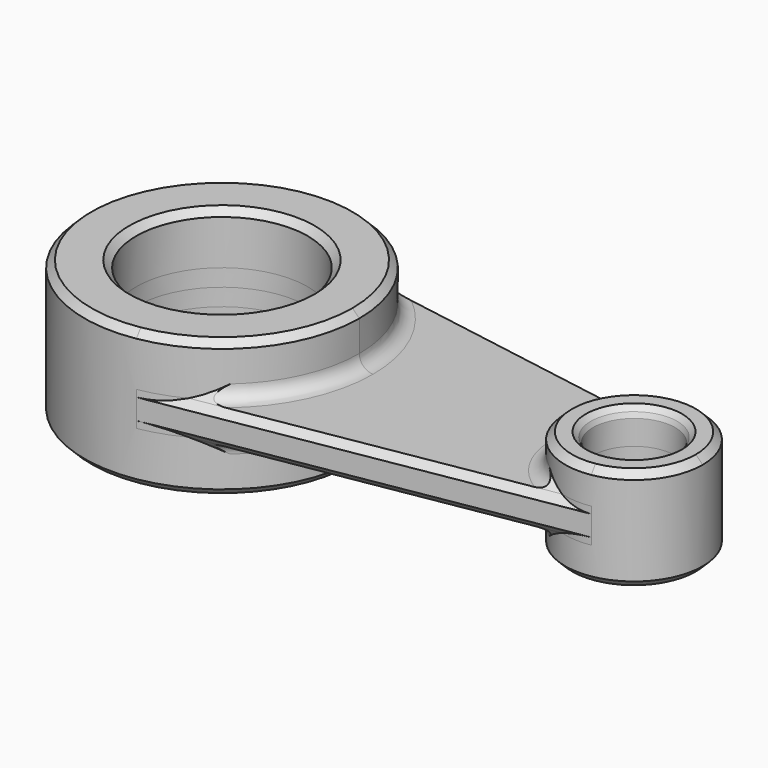
from build123d import *

# Parameters (mm, degrees)
F0_R         = 12.5
F0_R_2       = 6
F1_DEPTH     = 2.5
F2_DEPTH     = 7.5
F3_DEPTH     = 10
F4_SIZE      = 1
F5_SIZE      = 1
F6_SIZE      = 1
F7_SIZE      = 1
F8_T4_DEPTH  = 74.5908957588
F8_S5_R      = 20
F8_T6_DEPTH  = 39
F8_S7_R      = 10
F8_T8_DEPTH  = 39
F8_T12_DEPTH = 74.5908957588
F8_S13_R     = 20
F8_T14_DEPTH = 39
F8_S15_R     = 10
F8_T16_DEPTH = 39
F8_T20_DEPTH = 74.5908957588
F8_S21_R     = 20
F8_T22_DEPTH = 39
F8_S23_R     = 10
F8_T24_DEPTH = 39
F8_T28_DEPTH = 74.5908957588
F8_S29_R     = 20
F8_T30_DEPTH = 39
F8_S31_R     = 10
F8_T32_DEPTH = 39
F9_T4_ANGLE  = 67.9417369476
F9_T9_ANGLE  = 67.9417369476
F9_T14_ANGLE = 170.4473240821
F9_T20_ANGLE = 67.9417369476
F9_T25_ANGLE = 67.9417369476
F9_T30_ANGLE = 170.4473240821


# Not quite as in the source:
# - a fillet or chamfer that OpenCascade refuses, or shapes differently, is made with other operations: its cross-section is extruded or revolved along the edge and cut away or added


with BuildPart() as f1:
    # F0 (on Top) → F1 (new body, symmetric)
    with BuildSketch(Plane.XY):
        with BuildLine():
            ThreePointArc((3.3333333333, -19.7202659437), (15.2752523165, -12.9099444874), (20, 0))
            ThreePointArc((20, 0), (15.2752523165, 12.9099444874), (3.3333333333, 19.7202659437))
            ThreePointArc((3.3333333333, 19.7202659437), (-20, 0), (3.3333333333, -19.7202659437))
        make_face()
        Circle(F0_R, mode=Mode.SUBTRACT)
        with BuildLine():
            ThreePointArc((3.3333333333, 19.7202659437), (15.2752523165, 12.9099444874), (20, 0))
            ThreePointArc((20, 0), (15.2752523165, -12.9099444874), (3.3333333333, -19.7202659437))
            Line((3.3333333333, -19.7202659437), (61.6666666667, -9.8601329718))
            ThreePointArc((61.6666666667, -9.8601329718), (50, 0), (61.6666666667, 9.8601329718))
            Line((61.6666666667, 9.8601329718), (3.3333333333, 19.7202659437))
        make_face()
        with BuildLine():
            ThreePointArc((70, 0), (67.6376261583, 6.4549722437), (61.6666666667, 9.8601329718))
            ThreePointArc((61.6666666667, 9.8601329718), (50, 0), (61.6666666667, -9.8601329718))
            ThreePointArc((61.6666666667, -9.8601329718), (67.6376261583, -6.4549722437), (70, 0))
        make_face()
        with Locations((60, 0)):
            Circle(F0_R_2, mode=Mode.SUBTRACT)
    extrude(amount=F1_DEPTH, both=True)

    # F0 (on Top) → F2 (join, symmetric)
    with BuildSketch(Plane.XY):
        with BuildLine():
            ThreePointArc((70, 0), (67.6376261583, 6.4549722437), (61.6666666667, 9.8601329718))
            ThreePointArc((61.6666666667, 9.8601329718), (50, 0), (61.6666666667, -9.8601329718))
            ThreePointArc((61.6666666667, -9.8601329718), (67.6376261583, -6.4549722437), (70, 0))
        make_face()
        with Locations((60, 0)):
            Circle(F0_R_2, mode=Mode.SUBTRACT)
    extrude(amount=F2_DEPTH, both=True)

    # F0 (on Top) → F3 (join, symmetric)
    with BuildSketch(Plane.XY):
        with BuildLine():
            ThreePointArc((3.3333333333, -19.7202659437), (15.2752523165, -12.9099444874), (20, 0))
            ThreePointArc((20, 0), (15.2752523165, 12.9099444874), (3.3333333333, 19.7202659437))
            ThreePointArc((3.3333333333, 19.7202659437), (-20, 0), (3.3333333333, -19.7202659437))
        make_face()
        Circle(F0_R, mode=Mode.SUBTRACT)
    extrude(amount=F3_DEPTH, both=True)

    # F4
    f4_edges = [f1.edges().sort_by_distance(p)[0] for p in [
        (-12.5, 0, 10),
        (54, 0, 7.5),
    ]]
    chamfer(f4_edges, length=F4_SIZE)

    # F5
    f5_edges = [f1.edges().sort_by_distance(p)[0] for p in [
        (-12.5, 0, -10),
        (54, 0, 0),
        (66, 0, -1.25),
        (54, 0, -2.5),
        (66, 0, 1.25),
        (54, 0, 2.5),
        (66, 0, -5),
        (54, 0, -7.5),
    ]]
    chamfer(f5_edges, length=F5_SIZE)

    # F6
    f6_edges = [f1.edges().sort_by_distance(p)[0] for p in [
        (-20, 0, -10),
        (50, 0, -7.5),
    ]]
    chamfer(f6_edges, length=F6_SIZE)

    # F7
    f7_edges = [f1.edges().sort_by_distance(p)[0] for p in [
        (-20, 0, 10),
        (50, 0, 7.5),
    ]]
    chamfer(f7_edges, length=F7_SIZE)

    # F8: chamfer of 1 on 5 edges, made by hand


with BuildPart() as f8_tool2:
    # F8_s3 → F8_t4 (new body)
    with BuildSketch(Plane(origin=(65.9404742002, -11.1459744658, 0), x_dir=(0, 0, 1), z_dir=(-0.9860132972, 0.1666666667, 0))):
        Polygon((2.5, 19), (1.5, 20), (2.5, 20), align=None)
    extrude(amount=F8_T4_DEPTH)

    # F8_s5 → F8_t6 (cut, symmetric)
    with BuildSketch(Plane.XY.offset(2)):
        Circle(F8_S5_R)
    extrude(amount=F8_T6_DEPTH, both=True, mode=Mode.SUBTRACT)

    # F8_s7 → F8_t8 (cut, symmetric)
    with BuildSketch(Plane.XY.offset(2)):
        with Locations((60, 0)):
            Circle(F8_S7_R)
    extrude(amount=F8_T8_DEPTH, both=True, mode=Mode.SUBTRACT)


with BuildPart() as f1_1:
    add(f1.part)

    # F8_t1: cut F8_tool2
    add(f8_tool2.part, mode=Mode.SUBTRACT)


with BuildPart() as f8_tool10:
    # F8_s11 → F8_t12 (new body)
    with BuildSketch(Plane(origin=(-7.6071408668, -1.285841494, 0), x_dir=(0, 0, 1), z_dir=(0.9860132972, 0.1666666667, 0))):
        Polygon((2.5, 19), (1.5, 20), (2.5, 20), align=None)
    extrude(amount=F8_T12_DEPTH)

    # F8_s13 → F8_t14 (cut, symmetric)
    with BuildSketch(Plane.XY.offset(2)):
        Circle(F8_S13_R)
    extrude(amount=F8_T14_DEPTH, both=True, mode=Mode.SUBTRACT)

    # F8_s15 → F8_t16 (cut, symmetric)
    with BuildSketch(Plane.XY.offset(2)):
        with Locations((60, 0)):
            Circle(F8_S15_R)
    extrude(amount=F8_T16_DEPTH, both=True, mode=Mode.SUBTRACT)


with BuildPart() as f1_2:
    add(f1_1.part)

    # F8_t9: cut F8_tool10
    add(f8_tool10.part, mode=Mode.SUBTRACT)


with BuildPart() as f8_tool18:
    # F8_s19 → F8_t20 (new body)
    with BuildSketch(Plane(origin=(-7.6071408668, -1.285841494, 0), x_dir=(0, 0, 1), z_dir=(0.9860132972, 0.1666666667, 0))):
        Polygon((-1.5, 20), (-2.5, 19), (-2.5, 20), align=None)
    extrude(amount=F8_T20_DEPTH)

    # F8_s21 → F8_t22 (cut, symmetric)
    with BuildSketch(Plane.XY.offset(-2)):
        Circle(F8_S21_R)
    extrude(amount=F8_T22_DEPTH, both=True, mode=Mode.SUBTRACT)

    # F8_s23 → F8_t24 (cut, symmetric)
    with BuildSketch(Plane.XY.offset(-2)):
        with Locations((60, 0)):
            Circle(F8_S23_R)
    extrude(amount=F8_T24_DEPTH, both=True, mode=Mode.SUBTRACT)


with BuildPart() as f1_3:
    add(f1_2.part)

    # F8_t17: cut F8_tool18
    add(f8_tool18.part, mode=Mode.SUBTRACT)


with BuildPart() as f8_tool26:
    # F8_s27 → F8_t28 (new body)
    with BuildSketch(Plane(origin=(65.9404742002, -11.1459744658, 0), x_dir=(0, 0, 1), z_dir=(-0.9860132972, 0.1666666667, 0))):
        Polygon((-1.5, 20), (-2.5, 19), (-2.5, 20), align=None)
    extrude(amount=F8_T28_DEPTH)

    # F8_s29 → F8_t30 (cut, symmetric)
    with BuildSketch(Plane.XY.offset(-2)):
        Circle(F8_S29_R)
    extrude(amount=F8_T30_DEPTH, both=True, mode=Mode.SUBTRACT)

    # F8_s31 → F8_t32 (cut, symmetric)
    with BuildSketch(Plane.XY.offset(-2)):
        with Locations((60, 0)):
            Circle(F8_S31_R)
    extrude(amount=F8_T32_DEPTH, both=True, mode=Mode.SUBTRACT)


with BuildPart() as f1_4:
    add(f1_3.part)

    # F8_t25: cut F8_tool26
    add(f8_tool26.part, mode=Mode.SUBTRACT)

    # F8_s33 → F8_t34 (revolve, cut)
    with BuildSketch(Plane.XZ):
        Polygon((66.2928932188, 6.7928932188), (66, 6.0857864376), (66, 6.5), align=None)
    revolve(axis=Axis((60, 0, 6.5), (0, 0, 1)), mode=Mode.SUBTRACT)

    # F9: fillet of radius 2 on 10 edges, made by hand


with BuildPart() as f9_tool2:
    # F9_s3 → F9_t4 (revolve)
    with BuildSketch(Plane.XZ):
        with BuildLine():
            ThreePointArc((20, 4.5), (20.5857864376, 3.0857864376), (22, 2.5))
            Line((22, 2.5), (22, 2.46))
            Line((22, 2.46), (19.96, 2.46))
            Line((19.96, 2.46), (19.96, 4.5))
            Line((19.96, 4.5), (20, 4.5))
        make_face()
    revolve(axis=Axis((0, 0, 2.5), (0, 0, -1)), revolution_arc=F9_T4_ANGLE)

    split(bisect_by=Plane(origin=(1.7916666667, -10.5996429447, 10.75), x_dir=(-0.9860132972, -0.1666666667, 0), z_dir=(-0.1178511302, 0.6972166888, -0.7071067812)), keep=Keep.TOP)


with BuildPart() as f1_5:
    add(f1_4.part)

    # F9_t1: union F9_tool2
    add(f9_tool2.part)


with BuildPart() as f9_tool7:
    # F9_s8 → F9_t9 (revolve)
    with BuildSketch(Plane(origin=(0, 0, 0), x_dir=(0, 0, 1), z_dir=(-0.9268024445, 0.3755492362, 0))):
        with BuildLine():
            ThreePointArc((4.5, 20), (3.0857864376, 20.5857864376), (2.5, 22))
            Line((2.5, 22), (2.46, 22))
            Line((2.46, 22), (2.46, 19.96))
            Line((2.46, 19.96), (4.5, 19.96))
            Line((4.5, 19.96), (4.5, 20))
        make_face()
    revolve(axis=Axis((0, 0, 2.5), (0, 0, -1)), revolution_arc=F9_T9_ANGLE)

    split(bisect_by=Plane(origin=(1.7916666667, 10.5996429447, 10.75), x_dir=(0.9860132972, -0.1666666667, 0), z_dir=(-0.1178511302, -0.6972166888, -0.7071067812)), keep=Keep.TOP)


with BuildPart() as f1_6:
    add(f1_5.part)

    # F9_t6: union F9_tool7
    add(f9_tool7.part)


with BuildPart() as f9_tool12:
    # F9_s13 → F9_t14 (revolve)
    with BuildSketch(Plane(origin=(59.5840033564, -4.9786288681, 0), x_dir=(0, 0, 1), z_dir=(0.9965273316, -0.0832663041, 0))):
        with BuildLine():
            ThreePointArc((2.5, 7.0040217561), (3.0857864376, 5.5898081937), (4.5, 5.0040217561))
            Line((4.5, 5.0040217561), (4.5, 4.9640217561))
            Line((4.5, 4.9640217561), (2.46, 4.9640217561))
            Line((2.46, 4.9640217561), (2.46, 7.0040217561))
            Line((2.46, 7.0040217561), (2.5, 7.0040217561))
        make_face()
    revolve(axis=Axis((60, 0, 2.5), (0, 0, -1)), revolution_arc=F9_T14_ANGLE)

    split(bisect_by=Plane(origin=(1.7916666667, 10.5996429447, 10.75), x_dir=(0.9860132972, -0.1666666667, 0), z_dir=(-0.1178511302, -0.6972166888, -0.7071067812)), keep=Keep.TOP)

    split(bisect_by=Plane(origin=(1.7916666667, -10.5996429447, 10.75), x_dir=(-0.9860132972, -0.1666666667, 0), z_dir=(-0.1178511302, 0.6972166888, -0.7071067812)), keep=Keep.TOP)


with BuildPart() as f1_7:
    add(f1_6.part)

    # F9_t11: union F9_tool12
    add(f9_tool12.part)


with BuildPart() as f9_tool18:
    # F9_s19 → F9_t20 (revolve)
    with BuildSketch(Plane(origin=(0, 0, 0), x_dir=(0, 0, 1), z_dir=(-0.9268024445, -0.3755492362, 0))):
        with BuildLine():
            ThreePointArc((-2.5, -22), (-3.0857864376, -20.5857864376), (-4.5, -20))
            Line((-4.5, -20), (-4.5, -19.96))
            Line((-4.5, -19.96), (-2.46, -19.96))
            Line((-2.46, -19.96), (-2.46, -22))
            Line((-2.46, -22), (-2.5, -22))
        make_face()
    revolve(axis=Axis((0, 0, -2.5), (0, 0, 1)), revolution_arc=F9_T20_ANGLE)

    split(bisect_by=Plane(origin=(1.7916666667, -10.5996429447, -10.75), x_dir=(-0.9860132972, -0.1666666667, 0), z_dir=(-0.1178511302, 0.6972166888, 0.7071067812)), keep=Keep.TOP)


with BuildPart() as f1_8:
    add(f1_7.part)

    # F9_t17: union F9_tool18
    add(f9_tool18.part)


with BuildPart() as f9_tool23:
    # F9_s24 → F9_t25 (revolve)
    with BuildSketch(Plane.XZ):
        with BuildLine():
            ThreePointArc((22, -2.5), (20.5857864376, -3.0857864376), (20, -4.5))
            Line((20, -4.5), (19.96, -4.5))
            Line((19.96, -4.5), (19.96, -2.46))
            Line((19.96, -2.46), (22, -2.46))
            Line((22, -2.46), (22, -2.5))
        make_face()
    revolve(axis=Axis((0, 0, -2.5), (0, 0, 1)), revolution_arc=F9_T25_ANGLE)

    split(bisect_by=Plane(origin=(1.7916666667, 10.5996429447, -10.75), x_dir=(0.9860132972, -0.1666666667, 0), z_dir=(-0.1178511302, -0.6972166888, 0.7071067812)), keep=Keep.TOP)


with BuildPart() as f1_9:
    add(f1_8.part)

    # F9_t22: union F9_tool23
    add(f9_tool23.part)


with BuildPart() as f9_tool28:
    # F9_s29 → F9_t30 (revolve)
    with BuildSketch(Plane(origin=(59.5840033564, 4.9786288681, 0), x_dir=(0, 0, 1), z_dir=(0.9965273316, 0.0832663041, 0))):
        with BuildLine():
            ThreePointArc((-2.5, -7.0040217561), (-3.0857864376, -5.5898081937), (-4.5, -5.0040217561))
            Line((-4.5, -5.0040217561), (-4.5, -4.9640217561))
            Line((-4.5, -4.9640217561), (-2.46, -4.9640217561))
            Line((-2.46, -4.9640217561), (-2.46, -7.0040217561))
            Line((-2.46, -7.0040217561), (-2.5, -7.0040217561))
        make_face()
    revolve(axis=Axis((60, 0, -2.5), (0, 0, 1)), revolution_arc=F9_T30_ANGLE)

    split(bisect_by=Plane(origin=(1.7916666667, -10.5996429447, -10.75), x_dir=(-0.9860132972, -0.1666666667, 0), z_dir=(-0.1178511302, 0.6972166888, 0.7071067812)), keep=Keep.TOP)

    split(bisect_by=Plane(origin=(1.7916666667, 10.5996429447, -10.75), x_dir=(0.9860132972, -0.1666666667, 0), z_dir=(-0.1178511302, -0.6972166888, 0.7071067812)), keep=Keep.TOP)


with BuildPart() as f1_10:
    add(f1_9.part)

    # F9_t27: union F9_tool28
    add(f9_tool28.part)


solid = f1_10.part
